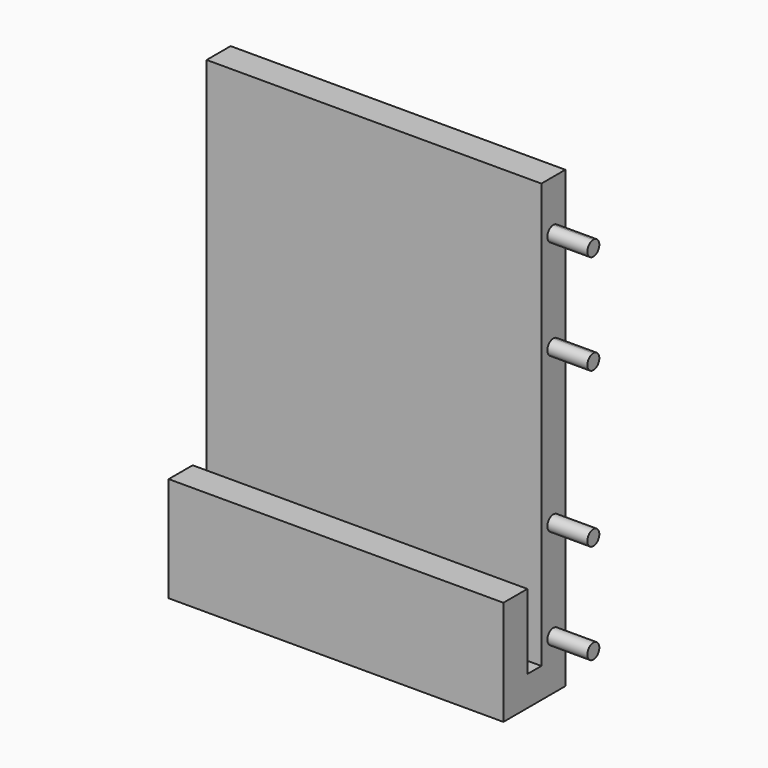
from build123d import *

# Parameters (mm, degrees)
F1_DEPTH = 67
F2_R     = 1.5
F3_DEPTH = 8
F4_R     = 1.875
F5_DEPTH = 9
F6_R     = 1.875
F7_DEPTH = 9
F8_R     = 1.875
F9_DEPTH = 9


# Not quite as in the source:
# - a feature names something its author has since deleted; it is built from what else it names


with BuildPart() as f1:
    # F0 (on Right) → F1 (new body)
    with BuildSketch(Plane.YZ):
        Polygon((14.9777059274, -37.1211464703), (14.9777059274, 53.8788535297), (8.9777059274, 53.8788535297), (8.9777059274, -31.1211464703), (5.4777059274, -31.1211464703), (5.4777059274, -16.1211464703), (-0.5222940726, -16.1211464703), (-0.5222940726, -37.1211464703), align=None)
    extrude(amount=F1_DEPTH)

    # F2 (on face) → F3 (join)
    with BuildSketch(Plane.YZ.offset(67)):
        with BuildLine():
            Line((11.9777059274, 43.8788535297), (11.9777059274, 45.3788535297))
            ThreePointArc((11.9777059274, 45.3788535297), (10.4777059274, 43.8788535297), (11.9777059274, 42.3788535297))
            Line((11.9777059274, 42.3788535297), (11.9777059274, 43.8788535297))
        make_face()
        with BuildLine():
            ThreePointArc((11.9777059274, 42.3788535297), (13.0383660992, 42.8181933579), (13.4777059274, 43.8788535297))
            ThreePointArc((13.4777059274, 43.8788535297), (13.0383660992, 44.9395137015), (11.9777059274, 45.3788535297))
            Line((11.9777059274, 45.3788535297), (11.9777059274, 43.8788535297))
            Line((11.9777059274, 43.8788535297), (11.9777059274, 42.3788535297))
        make_face()
        with BuildLine():
            ThreePointArc((13.4777059274, 23.8788535297), (13.0383660992, 24.9395137015), (11.9777059274, 25.3788535297))
            ThreePointArc((11.9777059274, 25.3788535297), (10.9170457557, 22.8181933579), (13.4777059274, 23.8788535297))
        make_face()
        with Locations((11.9777059274, -7.1211464703)):
            Circle(F2_R)
        with Locations((11.9777059274, -27.1211464703)):
            Circle(F2_R)
    extrude(amount=F3_DEPTH)

    # F4 (on face) → F5 (cut)
    with BuildSketch(Plane(origin=(0, 0, 0), x_dir=(0, -1, 0), z_dir=(-1, 0, 0))):
        with Locations((-18.4777059274, 23.8788535297)):
            Circle(F4_R)
        with Locations((-18.4777059274, 43.8788535297)):
            Circle(F4_R)
        with Locations((-18.4777059274, -7.1211464703)):
            Circle(F4_R)
        with Locations((-18.4777059274, -27.1211464703)):
            Circle(F4_R)
    extrude(amount=-F5_DEPTH, mode=Mode.SUBTRACT)

    # F6 (on face) → F7 (cut)
    with BuildSketch(Plane(origin=(0, 14.9777059274, 0), x_dir=(-1, 0, 0), z_dir=(0, 1, 0))):
        with Locations((-47, -34.1211464703)):
            Circle(F6_R)
        with Locations((-20, -34.1211464703)):
            Circle(F6_R)
    extrude(amount=-F7_DEPTH, mode=Mode.SUBTRACT)

    # F8 (on face) → F9 (cut)
    with BuildSketch(Plane(origin=(0, 0, 0), x_dir=(0, -1, 0), z_dir=(-1, 0, 0))):
        with BuildLine():
            ThreePointArc((-10.1027059274, 43.8788535297), (-10.6518807127, 45.2046787444), (-11.9777059274, 45.7538535297))
            Line((-11.9777059274, 45.7538535297), (-11.9777059274, 43.8788535297))
            Line((-11.9777059274, 43.8788535297), (-11.9777059274, 42.0038535297))
            ThreePointArc((-11.9777059274, 42.0038535297), (-10.6518807127, 42.553028315), (-10.1027059274, 43.8788535297))
        make_face()
        with BuildLine():
            ThreePointArc((-10.1027059274, 23.8788535297), (-10.6518807127, 25.2046787444), (-11.9777059274, 25.7538535297))
            ThreePointArc((-11.9777059274, 25.7538535297), (-13.3035311422, 22.553028315), (-10.1027059274, 23.8788535297))
        make_face()
        with BuildLine():
            Line((-11.9777059274, 43.8788535297), (-11.9777059274, 45.7538535297))
            ThreePointArc((-11.9777059274, 45.7538535297), (-13.8527059274, 43.8788535297), (-11.9777059274, 42.0038535297))
            Line((-11.9777059274, 42.0038535297), (-11.9777059274, 43.8788535297))
        make_face()
        with Locations((-11.9777059274, -27.1211464703)):
            Circle(F8_R)
        with Locations((-11.9777059274, -7.1211464703)):
            Circle(F8_R)
    extrude(amount=-F9_DEPTH, mode=Mode.SUBTRACT)


solid = f1.part
